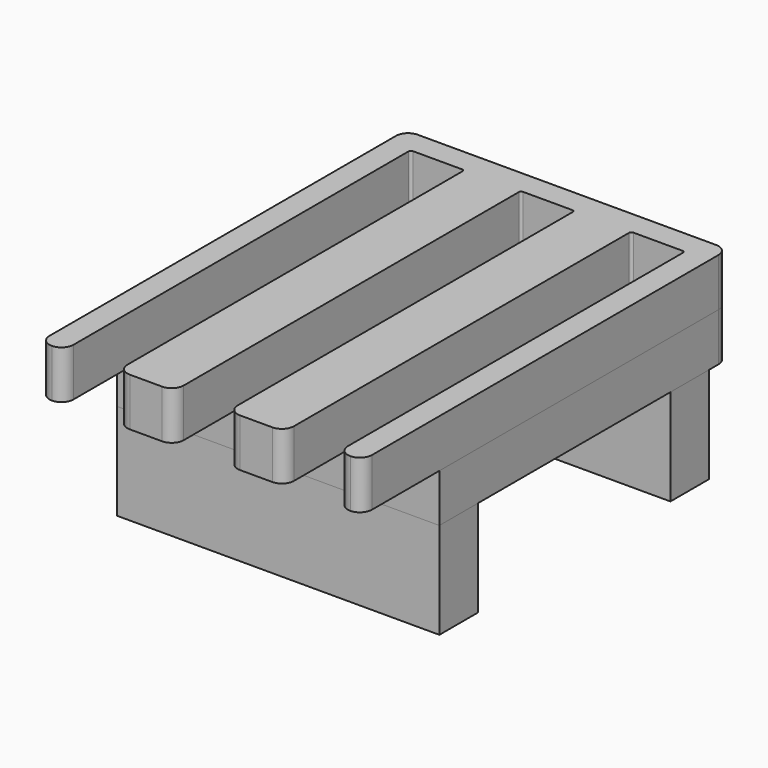
from build123d import *

# Parameters (mm, degrees)
F0_W     = 85.09
F0_H     = 95.25
F1_DEPTH = 12.7
F3_DEPTH = 12.7
F4_W     = 85.09
F4_H     = 12.7
F5_DEPTH = 25.4
F6_R     = 3.17499
F6_2_R   = 3.17499
F7_R     = 0.635


# Not quite as in the source:
# - a fillet or chamfer is up to 0.001 mm smaller than in the source, because OpenCascade refuses the exact size


with BuildPart() as f1:
    # F0 (on Top) → F1 (new body)
    with BuildSketch(Plane.XY):
        Rectangle(F0_W, F0_H)
    extrude(amount=F1_DEPTH)

    # F6#2 (radius 3.175 in the source; OpenCascade refuses exactly that, so slightly less here)
    f6_2_edges = [f1.edges().sort_by_distance(p)[0] for p in [
        (42.545, 47.625, 6.35),
        (-42.545, 47.625, 6.35),
    ]]
    fillet(f6_2_edges, radius=F6_2_R)


with BuildPart() as f3:
    # F2 (on face) → F3 (new body)
    with BuildSketch(Plane.XY.offset(12.7)):
        Polygon((21.971, -73.025), (21.971, 41.275), (36.195, 41.275), (36.195, -73.025), (42.545, -73.025), (42.545, 47.625), (-42.545, 47.625), (-42.545, -73.025), (-36.195, -73.025), (-36.195, 41.275), (-21.971, 41.275), (-21.971, -73.025), (-7.112, -73.025), (-7.112, 41.275), (7.112, 41.275), (7.112, -73.025), align=None)
    extrude(amount=F3_DEPTH)

    # F6 (radius 3.175 in the source; OpenCascade refuses exactly that, so slightly less here)
    f6_edges = [f3.edges().sort_by_distance(p)[0] for p in [
        (-36.195, -73.025, 19.05),
        (-42.545, -73.025, 19.05),
        (-21.971, -73.025, 19.05),
        (-7.112, -73.025, 19.05),
        (7.112, -73.025, 19.05),
        (21.971, -73.025, 19.05),
        (42.545, -73.025, 19.05),
        (42.545, 47.625, 19.05),
        (-42.545, 47.625, 19.05),
        (36.195, -73.025, 19.05),
    ]]
    fillet(f6_edges, radius=F6_R)

    # F7
    f7_edges = [f3.edges().sort_by_distance(p)[0] for p in [
        (-36.195, 41.275, 19.05),
        (-7.112, 41.275, 19.05),
        (21.971, 41.275, 19.05),
        (-21.971, 41.275, 19.05),
        (7.112, 41.275, 19.05),
        (36.195, 41.275, 19.05),
    ]]
    fillet(f7_edges, radius=F7_R)


with BuildPart() as f5:
    # F4 (on face) → F5 (new body)
    with BuildSketch(Plane(origin=(0, 0, 0), x_dir=(1, 0, 0), z_dir=(0, 0, -1))):
        with Locations((0, 41.275)):
            Rectangle(F4_W, F4_H)
    extrude(amount=F5_DEPTH)


with BuildPart() as f5b:
    # F4 (on face) → F5, piece 2 (new body)
    with BuildSketch(Plane(origin=(0, 0, 0), x_dir=(1, 0, 0), z_dir=(0, 0, -1))):
        with Locations((0, -34.925)):
            Rectangle(F4_W, F4_H)
    extrude(amount=F5_DEPTH)


solid = Compound([f1.part, f3.part, f5.part, f5b.part])
